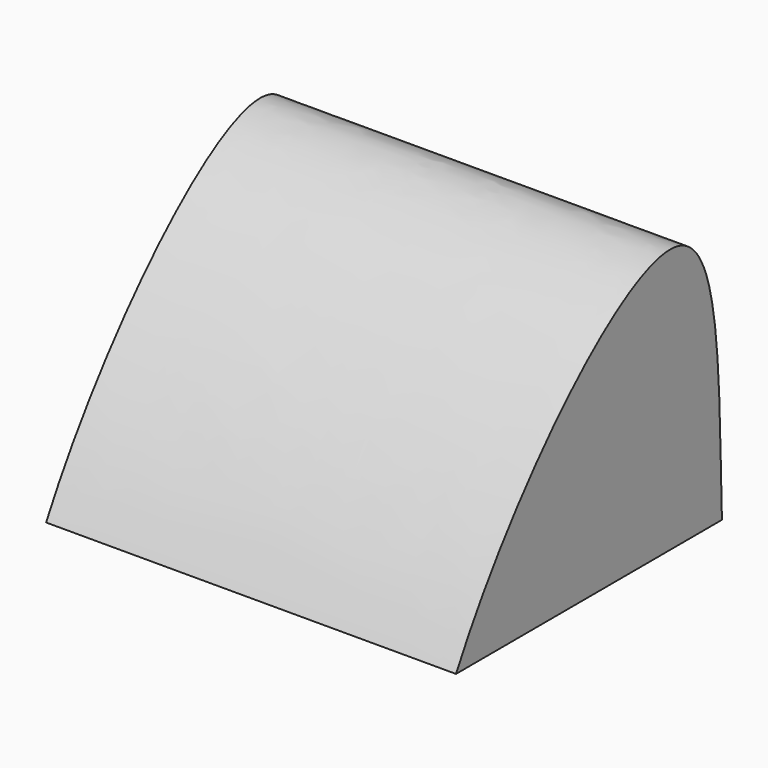
from build123d import *

# Parameters (mm, degrees)
F1_DEPTH = 148


with BuildPart() as f1:
    # F0 (on Right) → F1 (new body)
    with BuildSketch(Plane.YZ):
        with BuildLine():
            add(Edge.make_bspline(
                [(-101.1428560598, 0), (-74.4107142091, 50.4971072078), (20.5957118857, 144.8632694137), (17.4190876133, 42.7774296872), (18.8506282277, 0.1932075578)],
                knots=[0, 0, 0, 0, 0.5448244301, 0.9993125576, 0.9993125576, 0.9993125576, 0.9993125576], degree=3))
            Line((-101.1428560598, 0), (18.8506282277, 0.1932075578))
        make_face()
    extrude(amount=F1_DEPTH)


solid = f1.part
